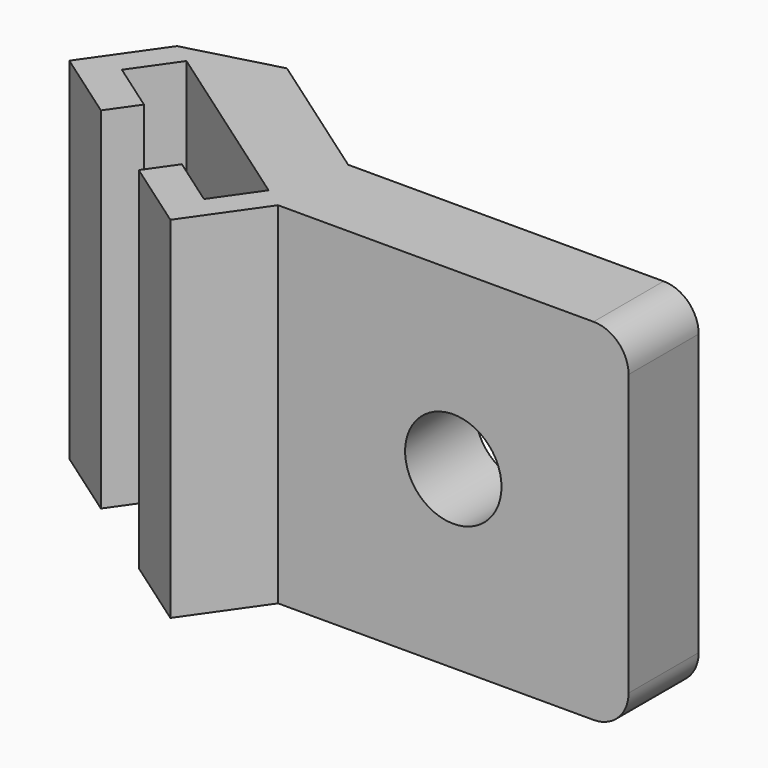
from build123d import *

# Parameters (mm, degrees)
F0_W      = 20
F0_H      = 5
F1_DEPTH  = 20
F2_R      = 2.75
F3_DEPTH  = 6.3
F3_FACE_R = 2.75
F4_DEPTH  = 6.5967602214
F5_R      = 2


# Not quite as in the source:
# - a feature names something its author has since deleted; it is built from what else it names


with BuildPart() as f1:
    # F0 (on Top) → F1 (new body)
    with BuildSketch(Plane.XY):
        Polygon((-10, -2.5), (-10, 2.5), (-17.9419796384, 8.0610340111), (-23.1064327086, 6.6772229816), (-21.8777046422, 5.8168583271), (-11.2287280664, -1.6396353455), align=None)
        Rectangle(F0_W, F0_H)
        Polygon((-21.8777046422, 5.8168583271), (-23.1064327086, 6.6772229816), (-25.9743148904, 2.5814627602), (-21.8785546689, -0.2864194216), (-20.7314017962, 1.351884667), (-23.5984339512, 3.3594021942), align=None)
        Polygon((-12.8678821818, -6.5957602214), (-10, -2.5), (-11.2287280664, -1.6396353455), (-12.9494573755, -4.0970914783), (-15.8164895305, -2.0895739511), (-16.9636424032, -3.7278780397), align=None)
    extrude(amount=F1_DEPTH)

    # F2 (on Front) → F3 (cut)
    with BuildSketch(Plane.XZ):
        with Locations((0, 10)):
            Circle(F2_R)
    extrude(amount=-F3_DEPTH, mode=Mode.SUBTRACT)

    # F2 (on Front) + F3_face (on face) → F4 (cut, through all)
    with BuildSketch(Plane.XZ):
        with Locations((0, 10)):
            Circle(F2_R)
    with BuildSketch(Plane(origin=(0, 0, 10), x_dir=(-1, 0, 0), z_dir=(0, 1, 0))):
        Circle(F3_FACE_R)
    extrude(amount=F4_DEPTH, dir=(0, -1, 0), mode=Mode.SUBTRACT)

    # F5
    f5_edges = [f1.edges().sort_by_distance(p)[0] for p in [
        (10, 0, 20),
        (10, 0, 0),
    ]]
    fillet(f5_edges, radius=F5_R)


solid = f1.part
